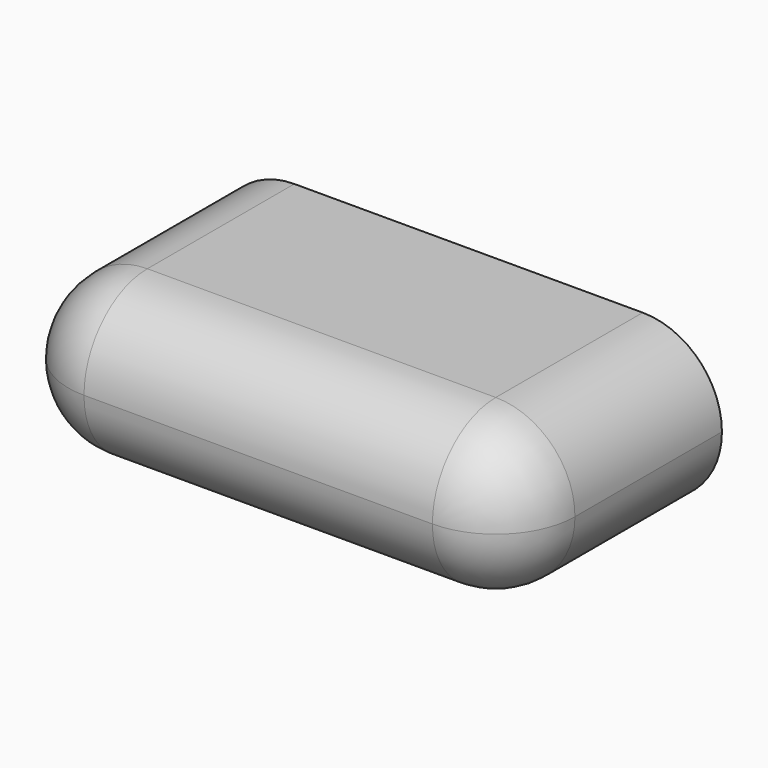
from build123d import *

# Parameters (mm, degrees)
F0_W     = 32
F0_H     = 10
F1_DEPTH = 16.6
F2_R     = 5
F3_R     = 4.99999
F4_R     = 4.99999


# Not quite as in the source:
# - a fillet or chamfer is up to 0.001 mm smaller than in the source, because OpenCascade refuses the exact size


with BuildPart() as f1:
    # F0 (on Front) → F1 (new body)
    with BuildSketch(Plane.XZ):
        Rectangle(F0_W, F0_H)
    extrude(amount=F1_DEPTH)

    # F2
    f2_edges = [f1.edges().sort_by_distance(p)[0] for p in [
        (16, -8.3, 5),
    ]]
    fillet(f2_edges, radius=F2_R)

    # F3 (radius 5 in the source; OpenCascade refuses exactly that, so slightly less here)
    f3_edges = [f1.edges().sort_by_distance(p)[0] for p in [
        (-16, -8.3, 5),
        (16, -8.3, -5),
        (-16, -8.3, -5),
    ]]
    fillet(f3_edges, radius=F3_R)

    # F4 (radius 5 in the source; OpenCascade refuses exactly that, so slightly less here)
    f4_edges = [f1.edges().sort_by_distance(p)[0] for p in [
        (-5e-06, -16.6, 5),
    ]]
    fillet(f4_edges, radius=F4_R)


solid = f1.part
